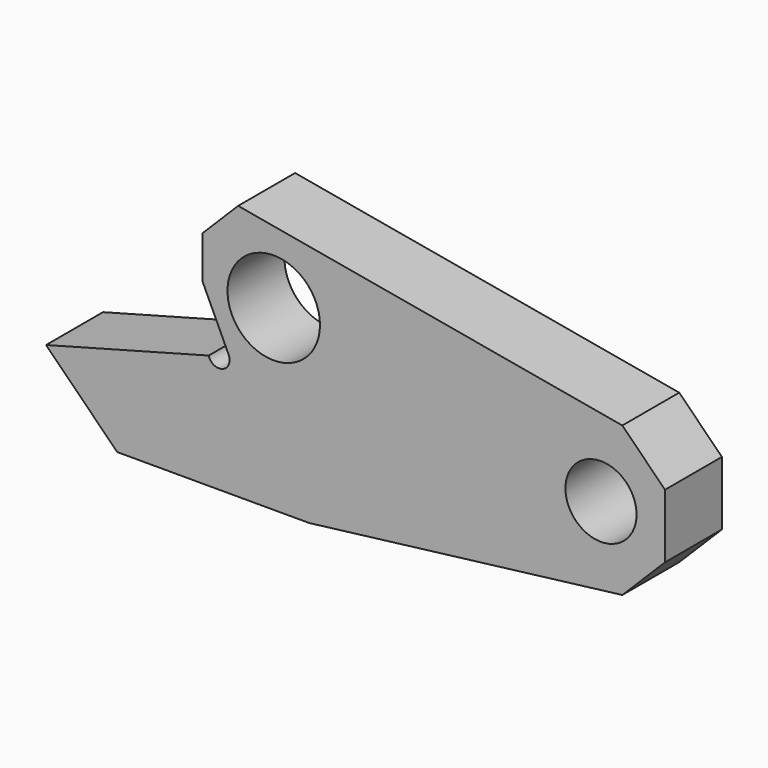
from build123d import *

# Parameters (mm, degrees)
F0_R     = 127
F0_R_2   = 165.1
F1_DEPTH = 254


# Not quite as in the source:
# - ends of sketch curves that miss each other by under 0.0002 mm in the source are joined


with BuildPart() as f1:
    # F0 (on Front) → F1 (new body)
    with BuildSketch(Plane.XZ):
        with BuildLine():
            Line((1314.5506856, -451.7077834), (1466.9506856, -299.3077834))
            Line((1466.9506856, -299.3077834), (1466.9506856, -71.2509878))
            Line((1466.9506856, -71.2509878), (1314.5506856, 81.1490122))
            Line((1314.5506856, 81.1490122), (-57.0493144, 325.4681832))
            Line((-57.0493144, 325.4681832), (-184.0493144, 198.4681832))
            Line((-184.0493144, 198.4681832), (-184.0493144, 46.0681832))
            Line((-184.0493144, 46.0681832), (-91.0235416, -153.4262362))
            ThreePointArc((-91.0235416, -153.4262362), (-112.5228808858, -205.3302952862), (-162.3556290296, -179.3889979113))
            Line((-162.3556290296, -179.3889979113), (-742.8493144, -334.9318168))
            Line((-742.8493144, -334.9318168), (-488.8493144, -588.9318168))
            Line((-488.8493144, -588.9318168), (196.9506856, -588.9318168))
            Line((196.9506856, -588.9318168), (1314.5506856, -451.7077834))
        make_face()
        with Locations((1238.3506856, -182.5318168)):
            Circle(F0_R, mode=Mode.SUBTRACT)
        with Locations((69.9506856, 46.0681832)):
            Circle(F0_R_2, mode=Mode.SUBTRACT)
    extrude(amount=F1_DEPTH)


solid = f1.part
